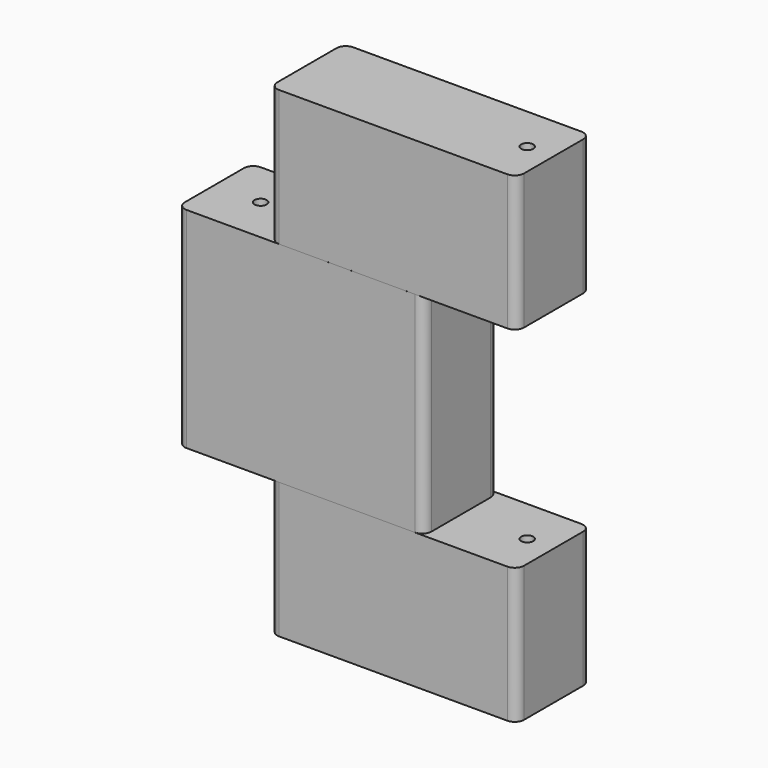
from build123d import *

# Parameters (mm, degrees)
F1_DEPTH     = 3.81
F3_START     = -0.000254
F3_DEPTH     = 3.81
F4_R         = 0.2501042953
F5_DEPTH     = 50.8
F6_T1_DEPTH  = 7.493
F6_T3_DEPTH  = 6.5405
F6_T5_DEPTH  = 7.493
F6_T7_DEPTH  = 6.5405
F6_T9_DEPTH  = 8.636
F6_T11_DEPTH = 10.541
F7_R         = 0.2501042953
F8_DEPTH     = 50.8


# Not quite as in the source:
# - a fillet or chamfer that OpenCascade refuses, or shapes differently, is made with other operations: its cross-section is extruded or revolved along the edge and cut away or added


with BuildPart() as f1:
    # F0 (on Front) → F1 (new body)
    with BuildSketch(Plane.XZ):
        Polygon((23.3729397243, -34.7344989846), (17.0229397243, -34.7344989846), (13.2129397243, -34.7344989846), (13.2129397243, -43.3704989846), (17.0229397243, -43.3704989846), (23.3729397243, -43.3704989846), align=None)
    extrude(amount=F1_DEPTH)

    # F2 (on face) → F3 (join)
    with BuildSketch(Plane.XZ.offset(3.81).offset(F3_START)):
        Polygon((27.1829397243, -29.1464989846), (17.0229397243, -29.1464989846), (17.0229397243, -34.7344989846), (23.3729397243, -34.7344989846), (27.1829397243, -34.7344989846), align=None)
        Polygon((27.1829397243, -43.3704989846), (23.3729397243, -43.3704989846), (17.0229397243, -43.3704989846), (17.0229397243, -48.9584989846), (27.1829397243, -48.9584989846), align=None)
    extrude(amount=-F3_DEPTH)

    # F4 (on face) → F5 (cut)
    with BuildSketch(Plane(origin=(0, 0, -48.9584989846), x_dir=(1, 0, 0), z_dir=(0, 0, -1))):
        with Locations((26.094635429, 1.904746)):
            Circle(F4_R)
    extrude(amount=-F5_DEPTH, mode=Mode.SUBTRACT)

    # F6: fillet of radius 0.381 on 12 edges, made by hand

    # F6_s2 → F6_t1 (cut)
    with BuildSketch(Plane.XY.offset(-35.6869989846)):
        with BuildLine():
            ThreePointArc((26.8019397243, -3.809746), (27.071347408, -3.6981536836), (27.1829397243, -3.428746))
            Line((27.1829397243, -3.428746), (27.1829397243, -3.809746))
            Line((27.1829397243, -3.809746), (26.8019397243, -3.809746))
        make_face()
        with BuildLine():
            ThreePointArc((27.1829397243, -0.380746), (27.071347408, -0.1113383164), (26.8019397243, 0.000254))
            Line((26.8019397243, 0.000254), (27.1829397243, 0.000254))
            Line((27.1829397243, 0.000254), (27.1829397243, -0.380746))
        make_face()
    extrude(amount=F6_T1_DEPTH, mode=Mode.SUBTRACT)

    # F6_s4 → F6_t3 (cut)
    with BuildSketch(Plane.XY.offset(-34.7344989846)):
        with BuildLine():
            ThreePointArc((17.4039397243, -3.809746), (17.1345320407, -3.6981536836), (17.0229397243, -3.428746))
            Line((17.0229397243, -3.428746), (17.0229397243, -3.809746))
            Line((17.0229397243, -3.809746), (17.4039397243, -3.809746))
        make_face()
        with BuildLine():
            ThreePointArc((17.0229397243, -0.380746), (17.1345320407, -0.1113383164), (17.4039397243, 0.000254))
            Line((17.4039397243, 0.000254), (17.0229397243, 0.000254))
            Line((17.0229397243, 0.000254), (17.0229397243, -0.380746))
        make_face()
    extrude(amount=F6_T3_DEPTH, mode=Mode.SUBTRACT)

    # F6_s6 → F6_t5 (cut)
    with BuildSketch(Plane.XY.offset(-49.9109989846)):
        with BuildLine():
            ThreePointArc((26.8019397243, -3.809746), (27.071347408, -3.6981536836), (27.1829397243, -3.428746))
            Line((27.1829397243, -3.428746), (27.1829397243, -3.809746))
            Line((27.1829397243, -3.809746), (26.8019397243, -3.809746))
        make_face()
        with BuildLine():
            ThreePointArc((27.1829397243, -0.380746), (27.071347408, -0.1113383164), (26.8019397243, 0.000254))
            Line((26.8019397243, 0.000254), (27.1829397243, 0.000254))
            Line((27.1829397243, 0.000254), (27.1829397243, -0.380746))
        make_face()
    extrude(amount=F6_T5_DEPTH, mode=Mode.SUBTRACT)

    # F6_s8 → F6_t7 (cut)
    with BuildSketch(Plane.XY.offset(-49.9109989846)):
        with BuildLine():
            ThreePointArc((17.0229397243, -3.428746), (17.1345320407, -3.6981536836), (17.4039397243, -3.809746))
            Line((17.4039397243, -3.809746), (17.0229397243, -3.809746))
            Line((17.0229397243, -3.809746), (17.0229397243, -3.428746))
        make_face()
        with BuildLine():
            ThreePointArc((17.0229397243, -0.380746), (17.1345320407, -0.1113383164), (17.4039397243, 0.000254))
            Line((17.4039397243, 0.000254), (17.0229397243, 0.000254))
            Line((17.0229397243, 0.000254), (17.0229397243, -0.380746))
        make_face()
    extrude(amount=F6_T7_DEPTH, mode=Mode.SUBTRACT)

    # F6_s10 → F6_t9 (cut)
    with BuildSketch(Plane.XY.offset(-43.3704989846)):
        with BuildLine():
            ThreePointArc((22.9919397243, -3.81), (23.261347408, -3.6984076836), (23.3729397243, -3.429))
            Line((23.3729397243, -3.429), (23.3729397243, -3.81))
            Line((23.3729397243, -3.81), (22.9919397243, -3.81))
        make_face()
        with BuildLine():
            ThreePointArc((22.9919397243, 0), (23.261347408, -0.1115923164), (23.3729397243, -0.381))
            Line((23.3729397243, -0.381), (23.3729397243, 0))
            Line((23.3729397243, 0), (22.9919397243, 0))
        make_face()
    extrude(amount=F6_T9_DEPTH, mode=Mode.SUBTRACT)

    # F6_s12 → F6_t11 (cut)
    with BuildSketch(Plane.XY.offset(-44.3229989846)):
        with BuildLine():
            ThreePointArc((13.2129397243, -3.429), (13.3245320407, -3.6984076836), (13.5939397243, -3.81))
            Line((13.5939397243, -3.81), (13.2129397243, -3.81))
            Line((13.2129397243, -3.81), (13.2129397243, -3.429))
        make_face()
        with BuildLine():
            ThreePointArc((13.5939397243, 0), (13.3245320407, -0.1115923164), (13.2129397243, -0.381))
            Line((13.2129397243, -0.381), (13.2129397243, 0))
            Line((13.2129397243, 0), (13.5939397243, 0))
        make_face()
    extrude(amount=F6_T11_DEPTH, mode=Mode.SUBTRACT)

    # F7 (on face) → F8 (cut)
    with BuildSketch(Plane(origin=(0, 0, -43.3704989846), x_dir=(1, 0, 0), z_dir=(0, 0, -1))):
        with Locations((15.1179397243, 1.904746)):
            Circle(F7_R)
    extrude(amount=-F8_DEPTH, mode=Mode.SUBTRACT)


solid = f1.part
